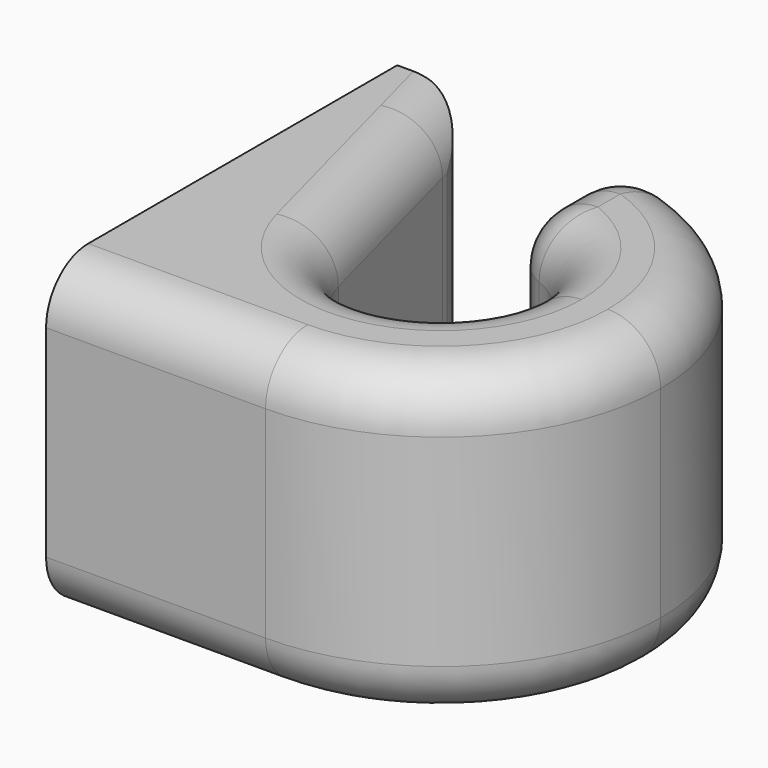
from build123d import *

# Parameters (mm, degrees)
F1_DEPTH = 7
F2_R     = 1.2


# Not quite as in the source:
# - a feature names something its author has since deleted; it is built from what else it names


with BuildPart() as f1:
    # F0 (on Top) → F1 (new body)
    with BuildSketch(Plane.XY):
        with BuildLine():
            Line((-5, -5), (0, -5))
            ThreePointArc((0, -5), (-3.5355339059, -3.5355339059), (-5, 0))
            Line((-5, 0), (-5, -5))
        make_face()
        with BuildLine():
            ThreePointArc((0, -5), (3.5355339059, -3.5355339059), (5, 0))
            ThreePointArc((5, 0), (3.5355339059, 3.5355339059), (0, 5))
            Line((0, 5), (0, 2))
            ThreePointArc((0, 2), (1.4142135624, 1.4142135624), (2, 0))
            ThreePointArc((2, 0), (0.2572150448, -1.9833911416), (-1.9338404207, -0.5101580414))
            Line((-1.9338404207, -0.5101580414), (-3.1027593412, 3.9208270136))
            ThreePointArc((-3.1027593412, 3.9208270136), (-4.5007664184, 2.177866306), (-5, 0))
            ThreePointArc((-5, 0), (-3.5355339059, -3.5355339059), (0, -5))
        make_face()
        with BuildLine():
            ThreePointArc((-5, 0), (-4.5007664184, 2.177866306), (-3.1027593412, 3.9208270136))
            Line((-3.1027593412, 3.9208270136), (-3.3874512792, 5))
            Line((-3.3874512792, 5), (-5, 5))
            Line((-5, 5), (-5, 0))
        make_face()
    extrude(amount=F1_DEPTH)

    # F2
    f2_edges = [f1.edges().sort_by_distance(p)[0] for p in [
        (1.584348, -1.220591, 0),
        (1.584348, -1.220591, 7),
        (5, 0, 0),
        (5, 0, 7),
        (0, 5, 3.5),
        (0, 2, 3.5),
        (0, 3.5, 7),
        (0, 3.5, 0),
        (-3.387451, 5, 3.5),
        (-2.5, -5, 0),
        (-2.5, -5, 7),
        (-2.660646, 2.244921, 0),
        (-2.660646, 2.244921, 7),
    ]]
    fillet(f2_edges, radius=F2_R)


solid = f1.part
